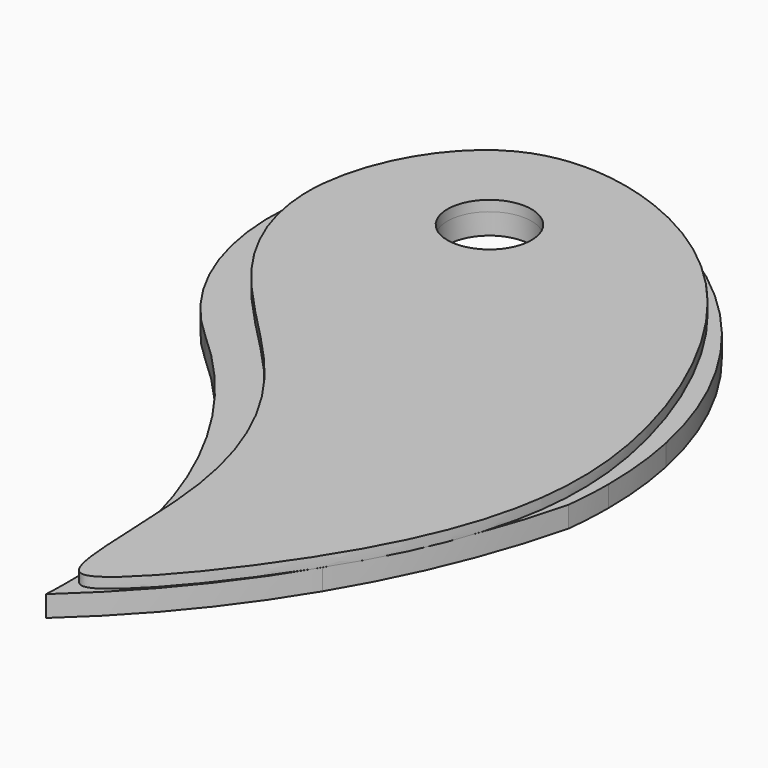
from build123d import *

# Parameters (mm, degrees)
F1_DEPTH = 1
F2_D     = 4
F4_DEPTH = 0.5
F5_D     = 4


# Not quite as in the source:
# - a feature names something its author has since deleted; it is built from what else it names


with BuildPart() as f1:
    # F0 (on Top) → F1 (new body)
    with BuildSketch(Plane.XY):
        with BuildLine():
            ThreePointArc((-4.6424048681, 3.80106262), (-2.0181143168, -5.6504172062), (6, 0))
            ThreePointArc((6, 0), (4.7435294982, 3.6740887169), (1.5003573667, 5.8093827359))
            ThreePointArc((1.5003573667, 5.8093827359), (-1.8645248851, 5.7029419559), (-4.6424048681, 3.80106262))
        make_face()
        with BuildLine():
            ThreePointArc((1.5003573667, 5.8093827359), (4.7435294982, 3.6740887169), (6, 0))
            ThreePointArc((6, 0), (-2.0181143168, -5.6504172062), (-4.6424048681, 3.80106262))
            ThreePointArc((-4.6424048681, 3.80106262), (-7.318751316, -4.7658127053), (-3.303978556, -12.7930029256))
            ThreePointArc((-3.303978556, -12.7930029256), (7.078551337, -15.5511771033), (15.5087052047, -8.8925768346))
            ThreePointArc((15.5087052047, -8.8925768346), (10.6056515013, 0.4603961331), (1.5003573667, 5.8093827359))
        make_face()
        with BuildLine():
            ThreePointArc((15.9087878687, -12.7930028931), (15.8085054873, -10.83255718), (15.5087052047, -8.8925768346))
            ThreePointArc((15.5087052047, -8.8925768346), (7.078551337, -15.5511771033), (-3.303978556, -12.7930029256))
            ThreePointArc((-3.303978556, -12.7930029256), (2.6233801475, -20.5925438503), (5.0986617771, -30.0709087245))
            ThreePointArc((5.0986617771, -30.0709087245), (8.7496291756, -27.7543175035), (11.7900910284, -24.6799477224))
            ThreePointArc((11.7900910284, -24.6799477224), (14.1459437512, -19.9966701457), (15.7798253656, -15.015348857))
            ThreePointArc((15.7798253656, -15.015348857), (15.8765201462, -13.9060452228), (15.9087878687, -12.7930028931))
        make_face()
        with BuildLine():
            ThreePointArc((11.7900910284, -24.6799477224), (8.7496291756, -27.7543175035), (5.0986617771, -30.0709087245))
            ThreePointArc((5.0986617771, -30.0709087245), (5.130455094, -30.7982515831), (5.1410558629, -31.5262117967))
            ThreePointArc((5.1410558629, -31.5262117967), (5.1333256528, -32.1478634275), (5.1101398029, -32.7691306185))
            ThreePointArc((5.1101398029, -32.7691306185), (8.7532813741, -28.9748900207), (11.7900910284, -24.6799477224))
        make_face()
    extrude(amount=-F1_DEPTH)

    # F2 (through all)
    with Locations(Plane.XY):
        with Locations((0, 0)):
            Hole(F2_D / 2)


with BuildPart() as f4:
    # F3 (on Top) → F4 (new body)
    with BuildSketch(Plane.XY):
        with BuildLine():
            add(Edge.make_bspline(
                [(-6.8962299265, -1.2546199141), (-6.626668451, 1.3725303486), (-3.5093090382, 7.0573512811), (5.9231715051, 5.0441838522), (11.9326397328, -1.2245690506), (15.1724840247, -9.1614223638), (15.7480132614, -16.2635016888), (12.8765786983, -23.9223462621), (6.9224077381, -31.3256150747), (4.7149088903, -31.6431390236), (5.3855520707, -22.1723322109), (1.4414285593, -14.15415947), (-5.2084107106, -8.7480398369), (-7.1589510611, -3.8151041102), (-6.8962299265, -1.2546199141)],
                knots=[0, 0, 0, 0, 0.0853995614, 0.1728482202, 0.263287429, 0.3522912072, 0.4323279076, 0.5225816841, 0.615421551, 0.6458614985, 0.7335064187, 0.8280664425, 0.9167675217, 1, 1, 1, 1], degree=3))
        make_face()
    extrude(amount=F4_DEPTH)

    # F5 (through all)
    with Locations(Plane(origin=(0, 0, 0), x_dir=(1, 0, 0), z_dir=(0, 0, -1))):
        with Locations((0, 0)):
            Hole(F5_D / 2)


solid = Compound([f1.part, f4.part])
